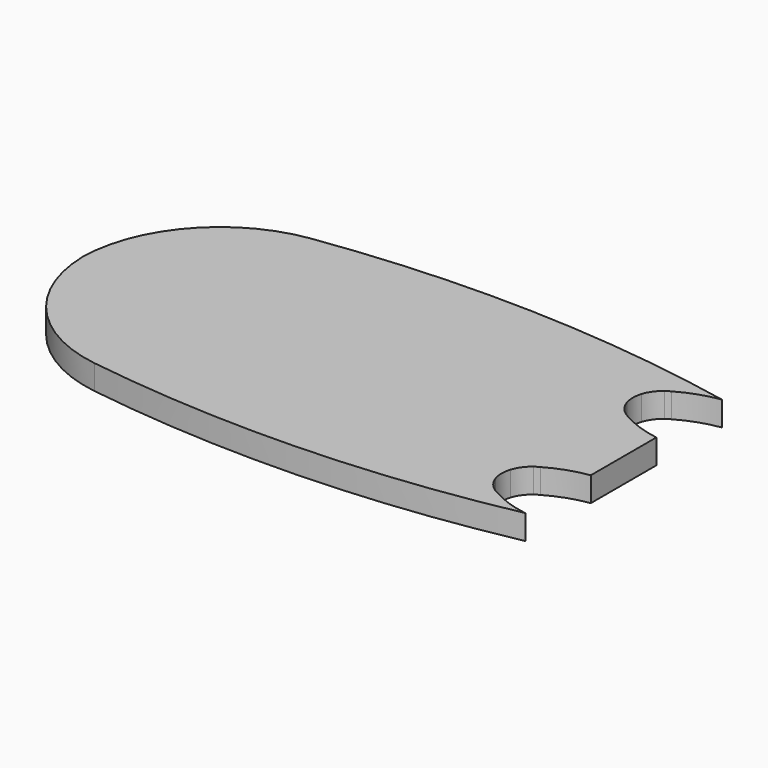
from build123d import *

# Parameters (mm, degrees)
F1_DEPTH    = 7.62
F2_T1_DEPTH = 231.4037837241


# Not quite as in the source:
# - a fillet or chamfer that OpenCascade refuses, or shapes differently, is made with other operations: its cross-section is extruded or revolved along the edge and cut away or added


with BuildPart() as f1:
    # F0 (on Top) → F1 (new body)
    with BuildSketch(Plane.XY):
        with BuildLine():
            ThreePointArc((64.7411976721, 47.7861853946), (-11.4588023279, 55.4061853946), (-87.6588023279, 47.7861853946))
            Line((-87.6588023279, 47.7861853946), (64.7411976721, 47.7861853946))
        make_face()
        with BuildLine():
            Line((-87.6588023279, -28.4138146054), (-87.6588023279, 47.7861853946))
            ThreePointArc((-87.6588023279, 47.7861853946), (-102.8988023279, 9.6861853946), (-87.6588023279, -28.4138146054))
        make_face()
        with BuildLine():
            Line((64.7411976721, 47.7861853946), (-87.6588023279, 47.7861853946))
            Line((-87.6588023279, 47.7861853946), (-87.6588023279, -28.4138146054))
            Line((-87.6588023279, -28.4138146054), (64.7411976721, -28.4138146054))
            ThreePointArc((64.7411976721, -28.4138146054), (58.4381171141, -26.858273051), (52.536175044, -24.1535339048))
            ThreePointArc((52.536175044, -24.1535339048), (51.7671122609, -23.7311786415), (51.0407896557, -23.2389419038))
            ThreePointArc((51.0407896557, -23.2389419038), (46.5861857996, -19.8140652327), (42.744152416, -15.7138146054))
            ThreePointArc((42.744152416, -15.7138146054), (46.5861857996, -11.6135639782), (51.0407896557, -8.188687307))
            ThreePointArc((51.0407896557, -8.188687307), (51.7671122609, -7.6964505693), (52.536175044, -7.2740953061))
            ThreePointArc((52.536175044, -7.2740953061), (58.4381171141, -4.5693561598), (64.7411976721, -3.0138146054))
            Line((64.7411976721, -3.0138146054), (64.7411976721, 22.3861853946))
            ThreePointArc((64.7411976721, 22.3861853946), (58.4381171141, 23.941726949), (52.536175044, 26.6464660952))
            ThreePointArc((52.536175044, 26.6464660952), (51.7671122609, 27.0688213585), (51.0407896557, 27.5610580962))
            ThreePointArc((51.0407896557, 27.5610580962), (46.5861857996, 30.9859347673), (42.744152416, 35.0861853946))
            ThreePointArc((42.744152416, 35.0861853946), (46.5861857996, 39.1864360218), (51.0407896557, 42.611312693))
            ThreePointArc((51.0407896557, 42.611312693), (51.7671122609, 43.1035494307), (52.536175044, 43.5259046939))
            ThreePointArc((52.536175044, 43.5259046939), (58.4381171141, 46.2306438402), (64.7411976721, 47.7861853946))
        make_face()
        with BuildLine():
            Line((64.7411976721, -28.4138146054), (-87.6588023279, -28.4138146054))
            ThreePointArc((-87.6588023279, -28.4138146054), (-11.4588023279, -36.0338146054), (64.7411976721, -28.4138146054))
        make_face()
        with BuildLine():
            ThreePointArc((51.0407896557, -23.2389419038), (49.0199759717, -21.171856557), (47.7230187251, -18.5883644093))
            Line((47.7230187251, -18.5883644093), (42.744152416, -15.7138146054))
            ThreePointArc((42.744152416, -15.7138146054), (46.5861857996, -19.8140652327), (51.0407896557, -23.2389419038))
        make_face()
        with BuildLine():
            Line((42.744152416, -15.7138146054), (47.7230187251, -18.5883644093))
            ThreePointArc((47.7230187251, -18.5883644093), (47.2726087596, -15.7138146054), (47.7230187251, -12.8392648016))
            Line((47.7230187251, -12.8392648016), (42.744152416, -15.7138146054))
        make_face()
        with BuildLine():
            ThreePointArc((51.0407896557, -8.188687307), (46.5861857996, -11.6135639782), (42.744152416, -15.7138146054))
            Line((42.744152416, -15.7138146054), (47.7230187251, -12.8392648016))
            ThreePointArc((47.7230187251, -12.8392648016), (49.0199759717, -10.2557726539), (51.0407896557, -8.188687307))
        make_face()
        with BuildLine():
            Line((42.744152416, 35.0861853946), (47.7230187251, 37.9607351984))
            ThreePointArc((47.7230187251, 37.9607351984), (49.0199759717, 40.5442273461), (51.0407896557, 42.611312693))
            ThreePointArc((51.0407896557, 42.611312693), (46.5861857996, 39.1864360218), (42.744152416, 35.0861853946))
        make_face()
        with BuildLine():
            ThreePointArc((47.7230187251, 32.2116355907), (47.2726087596, 35.0861853946), (47.7230187251, 37.9607351984))
            Line((47.7230187251, 37.9607351984), (42.744152416, 35.0861853946))
            Line((42.744152416, 35.0861853946), (47.7230187251, 32.2116355907))
        make_face()
        with BuildLine():
            Line((47.7230187251, 32.2116355907), (42.744152416, 35.0861853946))
            ThreePointArc((42.744152416, 35.0861853946), (46.5861857996, 30.9859347673), (51.0407896557, 27.5610580962))
            ThreePointArc((51.0407896557, 27.5610580962), (49.0199759717, 29.628143443), (47.7230187251, 32.2116355907))
        make_face()
    extrude(amount=F1_DEPTH)

    # F2: fillet of radius 43.18 on 2 edges, made by hand

    # F2_s2 → F2_t1 (cut)
    with BuildSketch(Plane.XY.offset(-111.891891862)):
        with BuildLine():
            ThreePointArc((-102.7512263975, 13.7215151075), (-93.3157996924, -16.5173565237), (-65.7822764709, -32.1801063989))
            ThreePointArc((-65.7822764709, -32.1801063989), (-76.7477031003, -30.4547410024), (-87.6588023279, -28.4138146054))
            ThreePointArc((-87.6588023279, -28.4138146054), (-99.6630733138, -8.9429787444), (-102.7512263975, 13.7215151075))
        make_face()
        with BuildLine():
            ThreePointArc((-65.7822764709, 51.552477188), (-93.3157996924, 35.8897273129), (-102.7512263975, 5.6508556816))
            ThreePointArc((-102.7512263975, 5.6508556816), (-99.6630733138, 28.3153495335), (-87.6588023279, 47.7861853946))
            ThreePointArc((-87.6588023279, 47.7861853946), (-76.7477031003, 49.8271117916), (-65.7822764709, 51.552477188))
        make_face()
    extrude(amount=F2_T1_DEPTH, mode=Mode.SUBTRACT)


solid = f1.part
